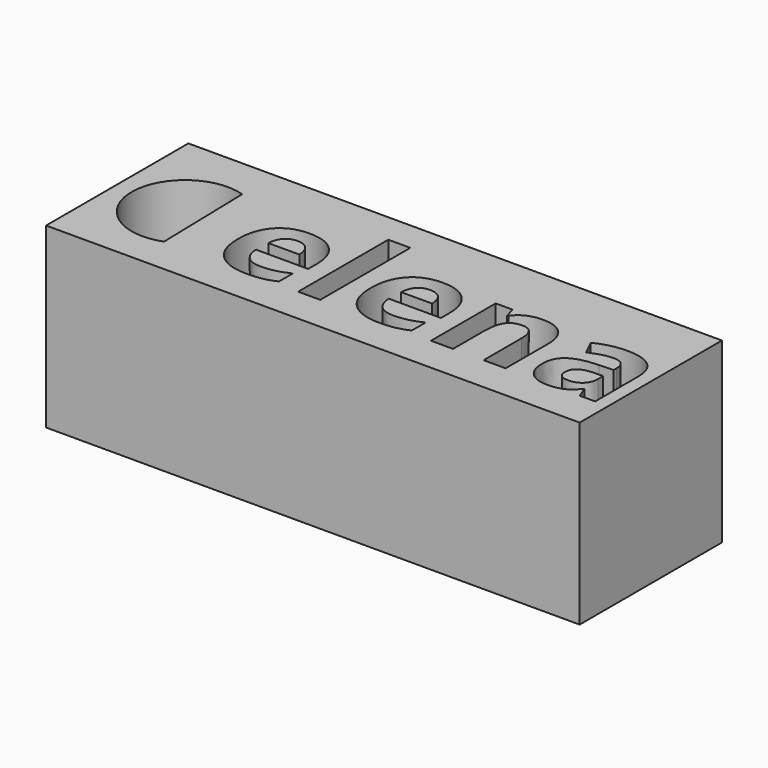
from build123d import *

# Parameters (mm, degrees)
F0_W         = 76.2
F0_H         = 25.4
F1_DEPTH     = 25.4
F4_DEPTH     = 25.4
F2_TEXT_SIZE = 21.1666666667
F5_DEPTH     = 25.4


# Not quite as in the source:
# - Text() gives the source's letters only with a copy of the font that has no kerning and outlines rounded to 1/6400 em; it was checked with that copy


with BuildPart() as f1:
    # F0 (on Top) → F1 (new body)
    with BuildSketch(Plane.XY):
        with Locations((38.1, -12.7)):
            Rectangle(F0_W, F0_H)
    extrude(amount=F1_DEPTH)

    # F3 (on Top) → F4 (cut)
    with BuildSketch(Plane.XY):
        with BuildLine():
            Line((12.7, -20.2246771944), (12.3577167095, -5.8488101333))
            ThreePointArc((12.3577167095, -5.8488101333), (2.3880996063, -13.2781908237), (12.7, -20.2246771944))
        make_face()
    extrude(amount=F4_DEPTH, mode=Mode.SUBTRACT)

    # F2 (on face) → F5 (cut)
    with BuildSketch(Plane.XY.offset(25.4)):
        with Locations((17.78, -20.32)):
            Text('elena', F2_TEXT_SIZE, font='Open Sans', font_style=FontStyle.BOLD, text_align=(TextAlign.LEFT, TextAlign.BOTTOM))
    extrude(amount=-F5_DEPTH, mode=Mode.SUBTRACT)


solid = f1.part
